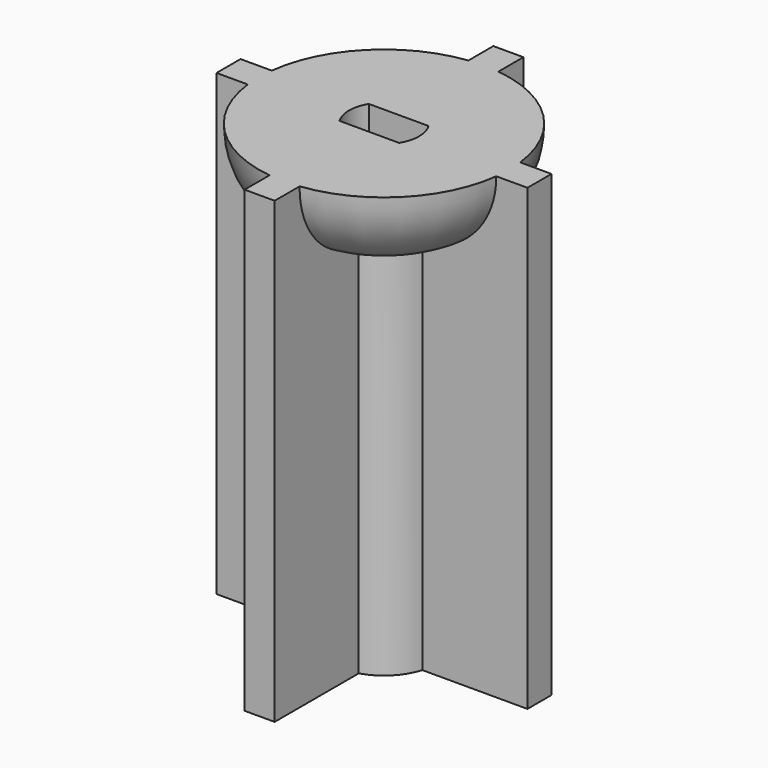
from build123d import *

# Parameters (mm, degrees)
F1_DEPTH     = 25
F3_DEPTH     = 7
F6_DEPTH     = 5
F7_DEPTH     = 2.5
F8_T4_ANGLE  = 265.6355670682
F8_T10_ANGLE = 265.6355670682
F8_T16_ANGLE = 265.6355670682
F8_T22_ANGLE = 265.6355670682
F8_T28_ANGLE = 265.6355670682
F8_T34_ANGLE = 265.6355670682
F8_T40_ANGLE = 265.6355670681
F8_T46_ANGLE = 265.6355670681
F8_T52_ANGLE = 265.6355670681
F8_T58_ANGLE = 265.6355670682
F8_T64_ANGLE = 265.6355670682
F8_T70_ANGLE = 265.6355670682


# Not quite as in the source:
# - a fillet or chamfer that OpenCascade refuses, or shapes differently, is made with other operations: its cross-section is extruded or revolved along the edge and cut away or added


with BuildPart() as f1:
    # F0 (on Top) → F1 (new body)
    with BuildSketch(Plane.XY):
        with BuildLine():
            ThreePointArc((3.0186917696, -0.9), (3.1170000862, -0.4547641838), (3.15, 0))
            ThreePointArc((3.15, 0), (3.1170000862, 0.4547641838), (3.0186917696, 0.9))
            ThreePointArc((3.0186917696, 0.9), (2.2273863607, 2.2273863607), (0.9, 3.0186917696))
            ThreePointArc((0.9, 3.0186917696), (0, 3.15), (-0.9, 3.0186917696))
            ThreePointArc((-0.9, 3.0186917696), (-2.2273863607, 2.2273863607), (-3.0186917696, 0.9))
            ThreePointArc((-3.0186917696, 0.9), (-3.15, 0), (-3.0186917696, -0.9))
            ThreePointArc((-3.0186917696, -0.9), (-2.2273863607, -2.2273863607), (-0.9, -3.0186917696))
            ThreePointArc((-0.9, -3.0186917696), (0, -3.15), (0.9, -3.0186917696))
            ThreePointArc((0.9, -3.0186917696), (2.2273863607, -2.2273863607), (3.0186917696, -0.9))
        make_face()
        with BuildLine():
            ThreePointArc((3.0186917696, 0.9), (3.1170000862, 0.4547641838), (3.15, 0))
            ThreePointArc((3.15, 0), (3.1170000862, -0.4547641838), (3.0186917696, -0.9))
            Line((3.0186917696, -0.9), (9.3186917696, -0.9))
            Line((9.3186917696, -0.9), (9.3186917696, 0.9))
            Line((9.3186917696, 0.9), (3.0186917696, 0.9))
        make_face()
        with BuildLine():
            ThreePointArc((-0.9, 3.0186917696), (0, 3.15), (0.9, 3.0186917696))
            Line((0.9, 3.0186917696), (0.9, 9.3186917696))
            Line((0.9, 9.3186917696), (-0.9, 9.3186917696))
            Line((-0.9, 9.3186917696), (-0.9, 3.0186917696))
        make_face()
        with BuildLine():
            Line((0.9, -9.3186917696), (0.9, -3.0186917696))
            ThreePointArc((0.9, -3.0186917696), (0, -3.15), (-0.9, -3.0186917696))
            Line((-0.9, -3.0186917696), (-0.9, -9.3186917696))
            Line((-0.9, -9.3186917696), (0.9, -9.3186917696))
        make_face()
        with BuildLine():
            ThreePointArc((-3.0186917696, -0.9), (-3.15, 0), (-3.0186917696, 0.9))
            Line((-3.0186917696, 0.9), (-9.3186917696, 0.9))
            Line((-9.3186917696, 0.9), (-9.3186917696, -0.9))
            Line((-9.3186917696, -0.9), (-3.0186917696, -0.9))
        make_face()
    extrude(amount=F1_DEPTH)

    # F2 (on face) → F3 (cut)
    with BuildSketch(Plane.XY.offset(25)):
        with BuildLine():
            ThreePointArc((1.788854382, -1.1), (2.020716977, -0.5715793024), (2.1, 0))
            ThreePointArc((2.1, 0), (2.020716977, 0.5715793024), (1.788854382, 1.1))
            Line((1.788854382, 1.1), (-1.788854382, 1.1))
            ThreePointArc((-1.788854382, 1.1), (-2.1, 0), (-1.788854382, -1.1))
            Line((-1.788854382, -1.1), (1.788854382, -1.1))
        make_face()
    extrude(amount=-F3_DEPTH, mode=Mode.SUBTRACT)

    # F5 (on face) → F6 (join)
    with BuildSketch(Plane.XY.offset(25)):
        with BuildLine():
            Line((-0.9, 3.0186917696), (-0.9, 7.4458041876))
            ThreePointArc((-0.9, 7.4458041876), (-5.3033008589, 5.3033008589), (-7.4458041876, 0.9))
            Line((-7.4458041876, 0.9), (-3.0186917696, 0.9))
            ThreePointArc((-3.0186917696, 0.9), (-2.2273863607, 2.2273863607), (-0.9, 3.0186917696))
        make_face()
        with BuildLine():
            ThreePointArc((-7.4458041876, -0.9), (-5.3033008589, -5.3033008589), (-0.9, -7.4458041876))
            Line((-0.9, -7.4458041876), (-0.9, -3.0186917696))
            ThreePointArc((-0.9, -3.0186917696), (-2.2273863607, -2.2273863607), (-3.0186917696, -0.9))
            Line((-3.0186917696, -0.9), (-7.4458041876, -0.9))
        make_face()
        with BuildLine():
            ThreePointArc((0.9, -7.4458041876), (5.3033008589, -5.3033008589), (7.4458041876, -0.9))
            Line((7.4458041876, -0.9), (3.0186917696, -0.9))
            ThreePointArc((3.0186917696, -0.9), (2.2273863607, -2.2273863607), (0.9, -3.0186917696))
            Line((0.9, -3.0186917696), (0.9, -7.4458041876))
        make_face()
        with BuildLine():
            Line((3.0186917696, 0.9), (7.4458041876, 0.9))
            ThreePointArc((7.4458041876, 0.9), (5.3033008589, 5.3033008589), (0.9, 7.4458041876))
            Line((0.9, 7.4458041876), (0.9, 3.0186917696))
            ThreePointArc((0.9, 3.0186917696), (2.2273863607, 2.2273863607), (3.0186917696, 0.9))
        make_face()
    extrude(amount=-F6_DEPTH)

    # F7 (add): a face of the model
    f7_faces = [f1.faces().sort_by_distance(p)[0] for p in [
        (0, 0, 0),
    ]]
    extrude(f7_faces, amount=F7_DEPTH)

    # F8: fillet of radius 5 on 4 edges, made by hand


with BuildPart() as f8_tool2:
    # F8_s3 → F8_t4 (revolve)
    with BuildSketch(Plane(origin=(0, 0, 0), x_dir=(0, 0, 1), z_dir=(0.0380776548, -0.9992747831, 0))):
        with BuildLine():
            ThreePointArc((20, -3.15), (21.6598434797, -6.2583240946), (24.9575699692, -7.5))
            Line((24.9575699692, -7.5), (20, -7.5))
            Line((20, -7.5), (20, -3.15))
        make_face()
    revolve(axis=Axis((0, 0, 20), (0, 0, 1)), revolution_arc=F8_T4_ANGLE)

    split(bisect_by=Plane.XZ.offset(-0.9), keep=Keep.BOTTOM)

    split(bisect_by=Plane.YZ.offset(0.9), keep=Keep.TOP)


with BuildPart() as f1_1:
    add(f1.part)

    # F8_t1: cut F8_tool2
    add(f8_tool2.part, mode=Mode.SUBTRACT)


with BuildPart() as f8_tool8:
    # F8_s9 → F8_t10 (revolve)
    with BuildSketch(Plane(origin=(0, 0, 0), x_dir=(0, 0, 1), z_dir=(0.0380776548, -0.9992747831, 0))):
        with BuildLine():
            ThreePointArc((20, -3.15), (21.6598434797, -6.2583240946), (24.9575699692, -7.5))
            Line((24.9575699692, -7.5), (20, -7.5))
            Line((20, -7.5), (20, -3.15))
        make_face()
    revolve(axis=Axis((0, 0, 20), (0, 0, 1)), revolution_arc=F8_T10_ANGLE)

    split(bisect_by=Plane.YZ.offset(-0.9), keep=Keep.BOTTOM)

    split(bisect_by=Plane.XZ.offset(-0.9), keep=Keep.BOTTOM)


with BuildPart() as f1_2:
    add(f1_1.part)

    # F8_t7: cut F8_tool8
    add(f8_tool8.part, mode=Mode.SUBTRACT)


with BuildPart() as f8_tool14:
    # F8_s15 → F8_t16 (revolve)
    with BuildSketch(Plane(origin=(0, 0, 0), x_dir=(0, 0, 1), z_dir=(0.0380776548, -0.9992747831, 0))):
        with BuildLine():
            ThreePointArc((20, -3.15), (21.6598434797, -6.2583240946), (24.9575699692, -7.5))
            Line((24.9575699692, -7.5), (20, -7.5))
            Line((20, -7.5), (20, -3.15))
        make_face()
    revolve(axis=Axis((0, 0, 20), (0, 0, 1)), revolution_arc=F8_T16_ANGLE)

    split(bisect_by=Plane.YZ.offset(-0.9), keep=Keep.BOTTOM)

    split(bisect_by=Plane.XZ.offset(0.9), keep=Keep.TOP)


with BuildPart() as f1_3:
    add(f1_2.part)

    # F8_t13: cut F8_tool14
    add(f8_tool14.part, mode=Mode.SUBTRACT)


with BuildPart() as f8_tool20:
    # F8_s21 → F8_t22 (revolve)
    with BuildSketch(Plane(origin=(0, 0, 0), x_dir=(0, 0, 1), z_dir=(-0.9992747831, -0.0380776548, 0))):
        with BuildLine():
            ThreePointArc((20, -3.15), (21.6598434797, -6.2583240946), (24.9575699692, -7.5))
            Line((24.9575699692, -7.5), (20, -7.5))
            Line((20, -7.5), (20, -3.15))
        make_face()
    revolve(axis=Axis((0, 0, 20), (0, 0, 1)), revolution_arc=F8_T22_ANGLE)

    split(bisect_by=Plane.XZ.offset(0.9), keep=Keep.TOP)

    split(bisect_by=Plane.YZ.offset(0.9), keep=Keep.TOP)


with BuildPart() as f1_4:
    add(f1_3.part)

    # F8_t19: cut F8_tool20
    add(f8_tool20.part, mode=Mode.SUBTRACT)


with BuildPart() as f8_tool26:
    # F8_s27 → F8_t28 (revolve)
    with BuildSketch(Plane(origin=(0, 0, 0), x_dir=(0, 0, 1), z_dir=(-0.9992747831, -0.0380776548, 0))):
        with BuildLine():
            ThreePointArc((20, -3.15), (21.6598434797, -6.2583240946), (24.9575699692, -7.5))
            Line((24.9575699692, -7.5), (20, -7.5))
            Line((20, -7.5), (20, -3.15))
        make_face()
    revolve(axis=Axis((0, 0, 20), (0, 0, 1)), revolution_arc=F8_T28_ANGLE)

    split(bisect_by=Plane.YZ.offset(0.9), keep=Keep.TOP)

    split(bisect_by=Plane.XZ.offset(-0.9), keep=Keep.BOTTOM)


with BuildPart() as f1_5:
    add(f1_4.part)

    # F8_t25: cut F8_tool26
    add(f8_tool26.part, mode=Mode.SUBTRACT)


with BuildPart() as f8_tool32:
    # F8_s33 → F8_t34 (revolve)
    with BuildSketch(Plane(origin=(0, 0, 0), x_dir=(0, 0, 1), z_dir=(-0.9992747831, -0.0380776548, 0))):
        with BuildLine():
            ThreePointArc((20, -3.15), (21.6598434797, -6.2583240946), (24.9575699692, -7.5))
            Line((24.9575699692, -7.5), (20, -7.5))
            Line((20, -7.5), (20, -3.15))
        make_face()
    revolve(axis=Axis((0, 0, 20), (0, 0, 1)), revolution_arc=F8_T34_ANGLE)

    split(bisect_by=Plane.XZ.offset(-0.9), keep=Keep.BOTTOM)

    split(bisect_by=Plane.YZ.offset(-0.9), keep=Keep.BOTTOM)


with BuildPart() as f1_6:
    add(f1_5.part)

    # F8_t31: cut F8_tool32
    add(f8_tool32.part, mode=Mode.SUBTRACT)


with BuildPart() as f8_tool38:
    # F8_s39 → F8_t40 (revolve)
    with BuildSketch(Plane(origin=(0, 0, 0), x_dir=(0, 0, 1), z_dir=(0.9992747831, 0.0380776548, 0))):
        with BuildLine():
            ThreePointArc((20, -3.15), (21.6598434797, -6.2583240946), (24.9575699692, -7.5))
            Line((24.9575699692, -7.5), (20, -7.5))
            Line((20, -7.5), (20, -3.15))
        make_face()
    revolve(axis=Axis((0, 0, 20), (0, 0, 1)), revolution_arc=F8_T40_ANGLE)

    split(bisect_by=Plane.YZ.offset(-0.9), keep=Keep.BOTTOM)

    split(bisect_by=Plane.XZ.offset(-0.9), keep=Keep.BOTTOM)


with BuildPart() as f1_7:
    add(f1_6.part)

    # F8_t37: cut F8_tool38
    add(f8_tool38.part, mode=Mode.SUBTRACT)


with BuildPart() as f8_tool44:
    # F8_s45 → F8_t46 (revolve)
    with BuildSketch(Plane(origin=(0, 0, 0), x_dir=(0, 0, 1), z_dir=(0.9992747831, 0.0380776548, 0))):
        with BuildLine():
            ThreePointArc((20, -3.15), (21.6598434797, -6.2583240946), (24.9575699692, -7.5))
            Line((24.9575699692, -7.5), (20, -7.5))
            Line((20, -7.5), (20, -3.15))
        make_face()
    revolve(axis=Axis((0, 0, 20), (0, 0, 1)), revolution_arc=F8_T46_ANGLE)

    split(bisect_by=Plane.XZ.offset(0.9), keep=Keep.TOP)

    split(bisect_by=Plane.YZ.offset(-0.9), keep=Keep.BOTTOM)


with BuildPart() as f1_8:
    add(f1_7.part)

    # F8_t43: cut F8_tool44
    add(f8_tool44.part, mode=Mode.SUBTRACT)


with BuildPart() as f8_tool50:
    # F8_s51 → F8_t52 (revolve)
    with BuildSketch(Plane(origin=(0, 0, 0), x_dir=(0, 0, 1), z_dir=(0.9992747831, 0.0380776548, 0))):
        with BuildLine():
            ThreePointArc((20, -3.15), (21.6598434797, -6.2583240946), (24.9575699692, -7.5))
            Line((24.9575699692, -7.5), (20, -7.5))
            Line((20, -7.5), (20, -3.15))
        make_face()
    revolve(axis=Axis((0, 0, 20), (0, 0, 1)), revolution_arc=F8_T52_ANGLE)

    split(bisect_by=Plane.XZ.offset(0.9), keep=Keep.TOP)

    split(bisect_by=Plane.YZ.offset(0.9), keep=Keep.TOP)


with BuildPart() as f1_9:
    add(f1_8.part)

    # F8_t49: cut F8_tool50
    add(f8_tool50.part, mode=Mode.SUBTRACT)


with BuildPart() as f8_tool56:
    # F8_s57 → F8_t58 (revolve)
    with BuildSketch(Plane(origin=(0, 0, 0), x_dir=(0, 0, 1), z_dir=(-0.0380776548, 0.9992747831, 0))):
        with BuildLine():
            ThreePointArc((24.9575699692, -7.5), (21.6598434797, -6.2583240946), (20, -3.15))
            Line((20, -3.15), (20, -7.5))
            Line((20, -7.5), (24.9575699692, -7.5))
        make_face()
    revolve(axis=Axis((0, 0, 20), (0, 0, 1)), revolution_arc=F8_T58_ANGLE)

    split(bisect_by=Plane.XZ.offset(0.9), keep=Keep.TOP)

    split(bisect_by=Plane.YZ.offset(-0.9), keep=Keep.BOTTOM)


with BuildPart() as f1_10:
    add(f1_9.part)

    # F8_t55: cut F8_tool56
    add(f8_tool56.part, mode=Mode.SUBTRACT)


with BuildPart() as f8_tool62:
    # F8_s63 → F8_t64 (revolve)
    with BuildSketch(Plane(origin=(0, 0, 0), x_dir=(0, 0, 1), z_dir=(-0.0380776548, 0.9992747831, 0))):
        with BuildLine():
            ThreePointArc((24.9575699692, -7.5), (21.6598434797, -6.2583240946), (20, -3.15))
            Line((20, -3.15), (20, -7.5))
            Line((20, -7.5), (24.9575699692, -7.5))
        make_face()
    revolve(axis=Axis((0, 0, 20), (0, 0, 1)), revolution_arc=F8_T64_ANGLE)

    split(bisect_by=Plane.XZ.offset(0.9), keep=Keep.TOP)

    split(bisect_by=Plane.YZ.offset(0.9), keep=Keep.TOP)


with BuildPart() as f1_11:
    add(f1_10.part)

    # F8_t61: cut F8_tool62
    add(f8_tool62.part, mode=Mode.SUBTRACT)


with BuildPart() as f8_tool68:
    # F8_s69 → F8_t70 (revolve)
    with BuildSketch(Plane(origin=(0, 0, 0), x_dir=(0, 0, 1), z_dir=(-0.0380776548, 0.9992747831, 0))):
        with BuildLine():
            ThreePointArc((24.9575699692, -7.5), (21.6598434797, -6.2583240946), (20, -3.15))
            Line((20, -3.15), (20, -7.5))
            Line((20, -7.5), (24.9575699692, -7.5))
        make_face()
    revolve(axis=Axis((0, 0, 20), (0, 0, 1)), revolution_arc=F8_T70_ANGLE)

    split(bisect_by=Plane.YZ.offset(0.9), keep=Keep.TOP)

    split(bisect_by=Plane.XZ.offset(-0.9), keep=Keep.BOTTOM)


with BuildPart() as f1_12:
    add(f1_11.part)

    # F8_t67: cut F8_tool68
    add(f8_tool68.part, mode=Mode.SUBTRACT)


solid = f1_12.part
